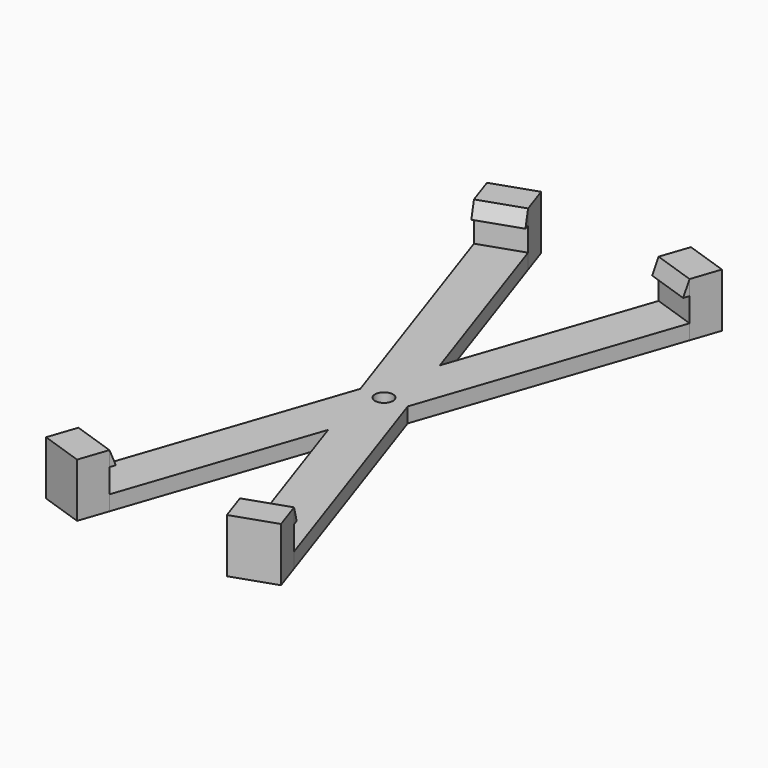
from build123d import *

# Parameters (mm, degrees)
F7_DEPTH = 5
F0_DEPTH = 18
F2_DEPTH = 15
F5_R     = 3
F8_DEPTH = 25


# Not quite as in the source:
# - a feature names something its author has since deleted; it is built from what else it names


with BuildPart() as f7:
    # F6 (on Top) → F7 (new body)
    with BuildSketch(Plane.XY):
        Polygon((0, -23.2909718978), (7.9219618343, -23.2909718978), (35.9808959381, 59.2037256741), (21.7798681683, 64.0339234217), (0, 0), align=None)
    extrude(amount=F7_DEPTH)

    # F6 (on Top) → F0 (join)
    with BuildSketch(Plane.XY):
        Polygon((21.7798681683, 64.0339234217), (35.9808959381, 59.2037256741), (39.2010277698, 68.6710775207), (25, 73.5012752683), align=None)
    extrude(amount=F0_DEPTH)

    # F1 (on face) → F2 (join, through all)
    with BuildSketch(Plane(origin=(0, 0, 0), x_dir=(-0.3220131832, -0.9467351847, 0), z_dir=(-0.9467351847, 0.3220131832, 0))):
        Polygon((-65.6365729928, 13), (-67.6365729928, 18), (-67.6365729928, 13), align=None)
    extrude(amount=-F2_DEPTH)

    # F3: F7 across face


with BuildPart() as f7_1:
    add(f7.part)
    add(f7.part.mirror(Plane(origin=(0, -11.6454859489, 2.5), x_dir=(0, -1, 0), z_dir=(-1, 0, 0))))

    # F4: F7 across face


with BuildPart() as f7_2:
    add(f7_1.part)
    add(f7_1.part.mirror(Plane(origin=(0, -23.2909718978, 2.5), x_dir=(1, 0, 0), z_dir=(0, -1, 0))))

    # F5 (on face) → F8 (cut)
    with BuildSketch(Plane.XY.offset(5)):
        with Locations((0, -23.2909718978)):
            Circle(F5_R)
    extrude(amount=-F8_DEPTH, mode=Mode.SUBTRACT)


solid = f7_2.part
